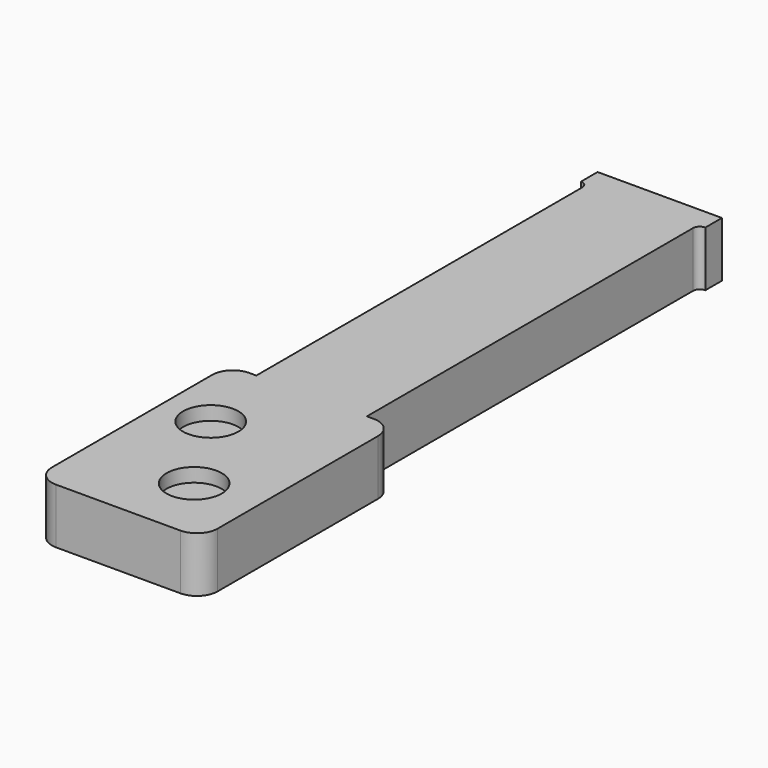
from build123d import *

# Parameters (mm, degrees)
F0_W     = 18
F0_H     = 8
F1_DEPTH = 3
F2_W     = 16
F2_H     = 8
F3_DEPTH = 60
F4_R     = 0.99999
F5_W     = 24
F5_H     = 8
F6_DEPTH = 35
F7_R     = 3
F8_R     = 4
F9_DEPTH = 2


# Not quite as in the source:
# - a fillet or chamfer is up to 0.001 mm smaller than in the source, because OpenCascade refuses the exact size


with BuildPart() as f1:
    # F0 (on Front) → F1 (new body)
    with BuildSketch(Plane.XZ):
        Rectangle(F0_W, F0_H)
    extrude(amount=F1_DEPTH)

    # F2 (on face) → F3 (join)
    with BuildSketch(Plane.XZ.offset(3)):
        Rectangle(F2_W, F2_H)
    extrude(amount=F3_DEPTH)

    # F4 (radius 1 in the source; OpenCascade refuses exactly that, so slightly less here)
    f4_edges = [f1.edges().sort_by_distance(p)[0] for p in [
        (-8, -3, 0),
        (8, -3, 0),
    ]]
    fillet(f4_edges, radius=F4_R)

    # F5 (on face) → F6 (join)
    with BuildSketch(Plane.XZ.offset(63)):
        Rectangle(F5_W, F5_H)
    extrude(amount=F6_DEPTH)

    # F7
    f7_edges = [f1.edges().sort_by_distance(p)[0] for p in [
        (-12, -63, 0),
        (-12, -98, 0),
        (12, -98, 0),
        (12, -63, 0),
    ]]
    fillet(f7_edges, radius=F7_R)

    # F8 (on face) → F9 (cut)
    with BuildSketch(Plane.XY.offset(4)):
        with Locations((-5, -75)):
            Circle(F8_R)
        with Locations((3, -88)):
            Circle(F8_R)
    extrude(amount=-F9_DEPTH, mode=Mode.SUBTRACT)


solid = f1.part
